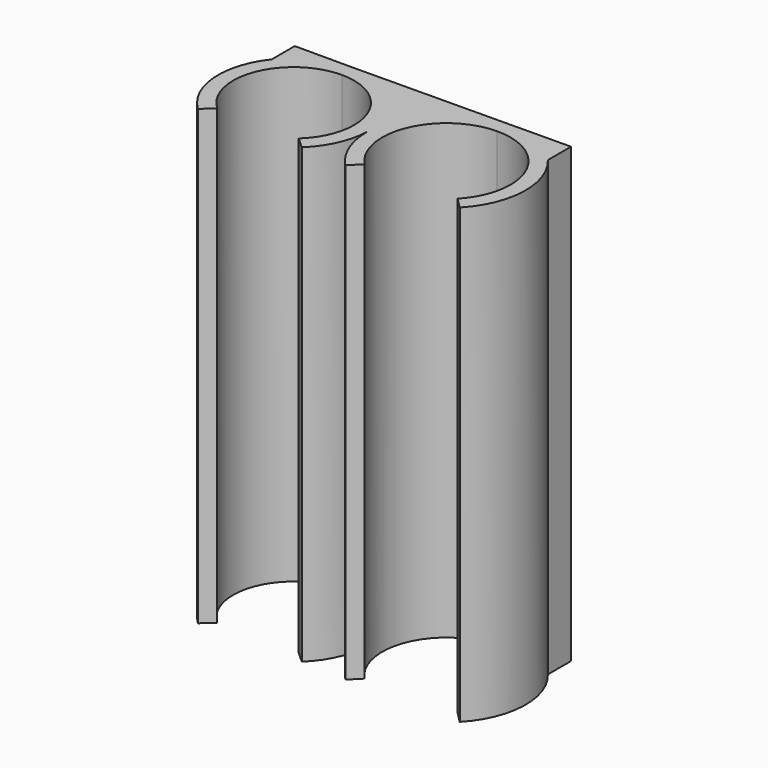
from build123d import *

# Parameters (mm, degrees)
F1_DEPTH    = 30
F2_T1_DEPTH = 30


# Not quite as in the source:
# - a fillet or chamfer that OpenCascade refuses, or shapes differently, is made with other operations: its cross-section is extruded or revolved along the edge and cut away or added
# - ends of sketch curves that miss each other by under 0.0002 mm in the source are joined
# - a feature names something its author has since deleted; it is built from what else it names


with BuildPart() as f1:
    # F0 (on Top) → F1 (new body)
    with BuildSketch(Plane.XY):
        with BuildLine():
            ThreePointArc((0.0090084839, 3.9999898559), (3.7308371777, 1.442516535), (2.6975556514, -2.9535052916))
            Line((2.6975556514, -2.9535052916), (3.4413844377, -3.6272404321))
            ThreePointArc((3.4413844377, -3.6272404321), (4.562894469, -2.0445033784), (4.9976265844, -0.1540406522))
            ThreePointArc((4.9976265844, -0.1540406522), (4.9982482299, -0.0770116198), (5, 0))
            ThreePointArc((5, 0), (4.4620948533, 2.2560384571), (2.964116192, 4.0266630354))
            Line((2.964116192, 4.0266630354), (0.0090084839, 3.9999898559))
        make_face()
        with BuildLine():
            ThreePointArc((-2.6975556514, -2.9535052916), (-3.7275789944, 1.4509151734), (0.0090084839, 3.9999898559))
            Line((0.0090084839, 3.9999898559), (2.964116192, 4.0266630354))
            ThreePointArc((2.964116192, 4.0266630354), (1.5599174374, 4.7504376207), (0, 5))
            ThreePointArc((0, 5), (-2.1802578035, 4.4996084175), (-3.9241225459, 3.0985903642))
            ThreePointArc((-3.9241225459, 3.0985903642), (-4.9871708669, -0.3579479625), (-3.4413844377, -3.6272404321))
            Line((-3.4413844377, -3.6272404321), (-2.6975556514, -2.9535052916))
        make_face()
        with BuildLine():
            ThreePointArc((0, 5), (1.5599174374, 4.7504376207), (2.964116192, 4.0266630354))
            Line((2.964116192, 4.0266630354), (7.1272566982, 4.0641686172))
            ThreePointArc((7.1272566982, 4.0641686172), (8.5825190892, 4.8210552933), (10.200330031, 5.0918944033))
            Line((10.200330031, 5.0918944033), (0, 5))
        make_face()
        with BuildLine():
            ThreePointArc((5, 0), (4.9982482299, -0.0770116198), (4.9976265844, -0.1540406522))
            ThreePointArc((4.9976265844, -0.1540406522), (4.9994066109, -0.0770294678), (5, 0))
        make_face()
        with BuildLine():
            ThreePointArc((5, 0), (4.9994066109, -0.0770294678), (4.9976265844, -0.1540406522))
            ThreePointArc((4.9976265844, -0.1540406522), (5.3752392401, -2.1129770441), (6.4564240892, -3.7895993711))
            Line((6.4564240892, -3.7895993711), (7.1655909773, -3.0842495499))
            ThreePointArc((7.1655909773, -3.0842495499), (6.3350165087, 1.5016234688), (10.2093385862, 4.0919349811))
            Line((10.2093385862, 4.0919349811), (7.1272566982, 4.0641686172))
            ThreePointArc((7.1272566982, 4.0641686172), (5.5962602055, 2.2767129418), (5, 0))
        make_face()
        with BuildLine():
            ThreePointArc((-3.9241225459, 3.0985903642), (-2.1802578035, 4.4996084175), (0, 5))
            Line((0, 5), (-3.9241225459, 5))
            Line((-3.9241225459, 5), (-3.9241225459, 3.0985903642))
        make_face()
        with BuildLine():
            ThreePointArc((10.200330031, 5.0918944033), (8.5825190892, 4.8210552933), (7.1272566982, 4.0641686172))
            Line((7.1272566982, 4.0641686172), (10.2093385862, 4.0919349811))
            Line((10.2093385862, 4.0919349811), (13.2914205601, 4.1197013458))
            ThreePointArc((13.2914205601, 4.1197013458), (11.8227579499, 4.8502464877), (10.200330031, 5.0918944033))
        make_face()
        with BuildLine():
            Line((14.2744146958, 5.1285976842), (10.200330031, 5.0918944033))
            ThreePointArc((10.200330031, 5.0918944033), (11.8227579499, 4.8502464877), (13.2914205601, 4.1197013458))
            ThreePointArc((13.2914205601, 4.1197013458), (13.8120129481, 3.6966683449), (14.2744146958, 3.2107074637))
            Line((14.2744146958, 3.2107074637), (14.2744146958, 5.1285976842))
        make_face()
        with BuildLine():
            Line((13.2914205601, 4.1197013458), (10.2093385862, 4.0919349811))
            ThreePointArc((10.2093385862, 4.0919349811), (14.145125137, 1.5368032872), (13.3296593654, -3.0842495499))
            Line((13.3296593654, -3.0842495499), (14.0388262535, -3.7895993711))
            ThreePointArc((14.0388262535, -3.7895993711), (15.4946546383, -0.3344761776), (14.2744146958, 3.2107074637))
            ThreePointArc((14.2744146958, 3.2107074637), (13.8120129481, 3.6966683449), (13.2914205601, 4.1197013458))
        make_face()
        with BuildLine():
            Line((7.1272566982, 4.0641686172), (2.964116192, 4.0266630354))
            ThreePointArc((2.964116192, 4.0266630354), (4.4620948533, 2.2560384571), (5, 0))
            ThreePointArc((5, 0), (5.5962602055, 2.2767129418), (7.1272566982, 4.0641686172))
        make_face()
    extrude(amount=F1_DEPTH)

    # F2: fillet of radius 1 on 1 edges, made by hand

    # F2_s2 → F2_t1 (join)
    with BuildSketch(Plane.XY):
        with BuildLine():
            ThreePointArc((0.0045042077, 5.0000405782), (-4.57e-08, 5.0000101446), (-0.0045043905, 5))
            Line((-0.0045043905, 5), (0, 5))
            Line((0, 5), (0.0045042077, 5.0000405782))
        make_face()
    extrude(amount=F2_T1_DEPTH)


solid = f1.part
